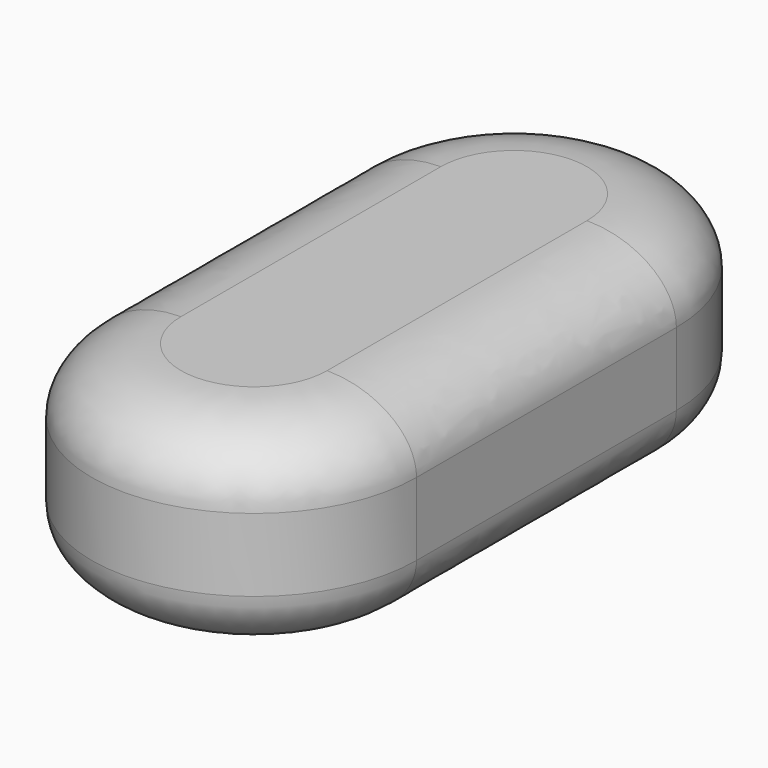
from build123d import *

# Parameters (mm, degrees)
F0_W     = 50.8
F0_H     = 31.75
F1_DEPTH = 101.6


# Not quite as in the source:
# - a feature names something its author has since deleted; it is built from what else it names
# - the program builds the solid bodies; features that only make, move or delete a surface that nothing else refers to are left out


with BuildPart() as f1:
    # F0 (on Front) → F1 (new body)
    with BuildSketch(Plane.XZ):
        with Locations((25.4, 15.875)):
            Rectangle(F0_W, F0_H)
    extrude(amount=-F1_DEPTH)

    # F5: sweep along a path in F2
    with BuildLine(Plane.XY.offset(31.75)) as f5_path:
        Line((50.8, 76.2), (50.8, 25.4))
        ThreePointArc((50.8, 25.4), (25.4, 0), (0, 25.4))
        Line((0, 25.4), (0, 76.2))
        ThreePointArc((0, 76.2), (25.4, 101.6), (50.8, 76.2))
    # F4 (on plane+point) → F5 (sweep, cut)
    with BuildSketch(Plane.XZ.offset(-25.4)):
        with BuildLine():
            Line((50.8, 21.59), (50.8, 31.75))
            Line((50.8, 31.75), (36.83, 31.75))
            add(Edge.make_bspline(
                [(50.8, 21.59), (50.8, 31.75), (36.83, 31.75)],
                knots=[0, 0, 0, 1.5707963268, 1.5707963268, 1.5707963268], degree=2, weights=[1, 0.7071067812, 1]))
        make_face()
        with BuildLine():
            Line((50.8, 0), (50.8, 10.16))
            add(Edge.make_bspline(
                [(36.83, 0), (50.8, 0), (50.8, 10.16)],
                knots=[4.7123889804, 4.7123889804, 4.7123889804, 6.2831853072, 6.2831853072, 6.2831853072], degree=2, weights=[1, 0.7071067812, 1]))
            Line((36.83, 0), (50.8, 0))
        make_face()
        Polygon((36.83, 31.75), (50.8, 31.75), (50.8, 21.59), (50.8, 10.16), (50.8, 0), (36.83, 0), (36.83, -19.05), (76.2, -19.05), (76.2, 10.16), (76.2, 21.59), (76.2, 50.8), (36.83, 50.8), align=None)
    sweep(path=f5_path.line, mode=Mode.SUBTRACT)


solid = f1.part
